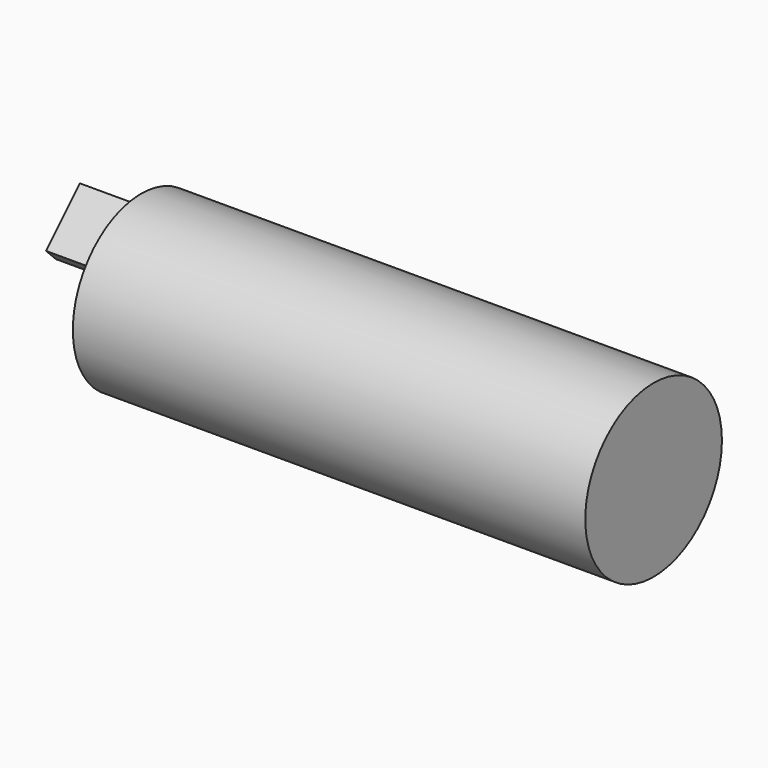
from build123d import *

# Parameters (mm, degrees)
F0_R     = 5
F1_DEPTH = 30
F2_E1_W  = 3.5025208565
F2_E1_H  = 5
F3_DEPTH = 1


with BuildPart() as f1:
    # F0 (on Right) → F1 (new body)
    with BuildSketch(Plane.YZ):
        Circle(F0_R)
    extrude(amount=F1_DEPTH)

    # F2_E1 (on explicit) → F3 (join)
    with BuildSketch(Plane(origin=(0, 0, 0), x_dir=(0, 0.7071067812, 0.7071067812), z_dir=(0, -0.7071067812, 0.7071067812))):
        with Locations((1.7512604282, 2.5)):
            Rectangle(F2_E1_W, F2_E1_H)
    extrude(amount=F3_DEPTH)


solid = f1.part
